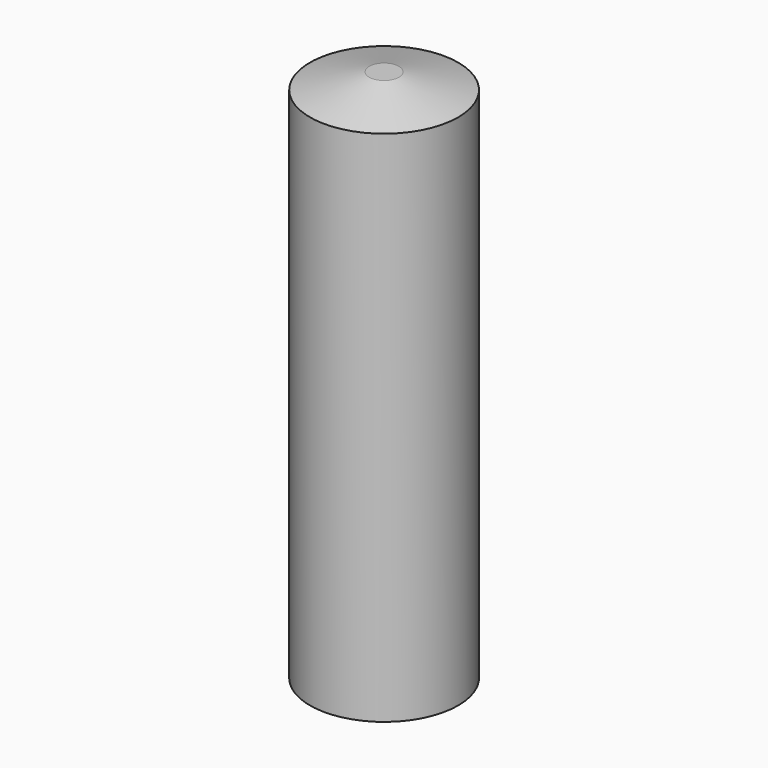
from build123d import *

# Parameters (mm, degrees)
F0_R     = 25
F1_DEPTH = 180
F2_SIZE2 = 5.3589838486
F2_SIZE  = 20
F4_D     = 17.5
F4_DEPTH = 60
F4_TIP   = 5.2575304165


with BuildPart() as f1:
    # F0 (on Top) → F1 (new body)
    with BuildSketch(Plane.XY):
        Circle(F0_R)
    extrude(amount=F1_DEPTH)

    # F2
    f2_edges = [f1.edges().sort_by_distance(p)[0] for p in [
        (-25, 0, 180),
    ]]
    f2_side = f1.faces().sort_by_distance((0, 0, 180))[0]
    chamfer(f2_edges, length=F2_SIZE, length2=F2_SIZE2, reference=f2_side)

    # F4
    with Locations(Plane(origin=(0, 0, 0), x_dir=(1, 0, 0), z_dir=(0, 0, -1))):
        with Locations((0, 0)):
            Hole(F4_D / 2, depth=F4_DEPTH)
            with Locations((0, 0, -(F4_DEPTH + F4_TIP / 2))):  # 118° drill point
                Cone(0, F4_D / 2, F4_TIP, mode=Mode.SUBTRACT)


solid = f1.part
